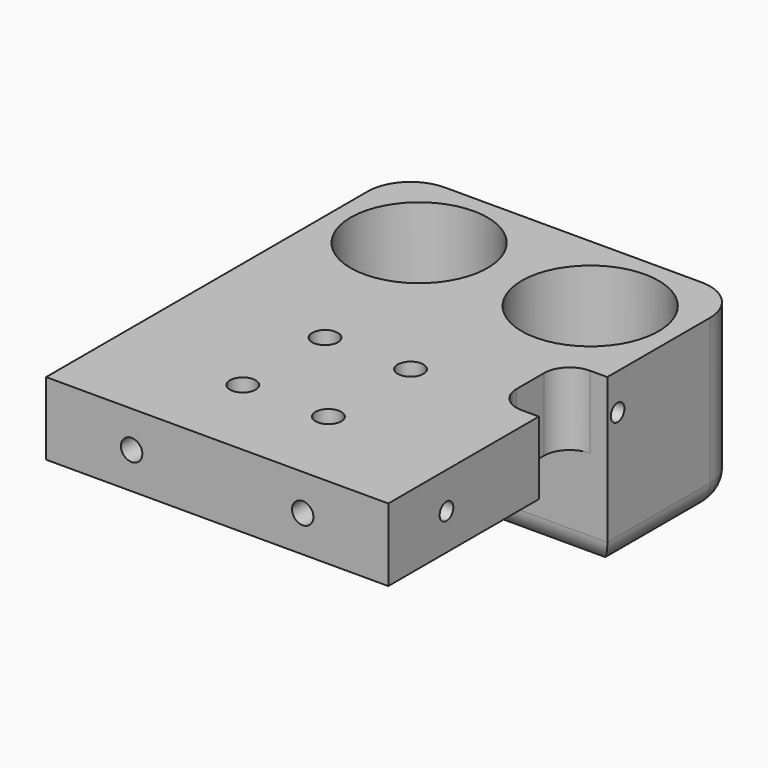
from build123d import *

# Parameters (mm, degrees)
F0_W          = 20
F0_H          = 20
F1_DEPTH      = 20
F2_D          = 3
F2_DEPTH      = 20
F2_TIP        = 0.9012909285
F3_D          = 16
F3_DEPTH      = 20
F3_TIP        = 4.8068849522
F4_W          = 40
F4_H          = 32
F4_R          = 1.5
F5_DEPTH      = 11.5
F7_D          = 2.5
F7_DEPTH      = 5
F7_TIP        = 0.7510757738
F8_R          = 5
F10_D         = 2.5
F10_DEPTH     = 5
F10_TIP       = 0.7510757738
F11_T1_DEPTH  = 22.5
F11_T3_DEPTH  = 55
F11_T5_DEPTH  = 30
F11_T8_ANGLE  = 90
F11_T10_ANGLE = 90
F13_W         = 5
F13_H         = 10
F14_DEPTH     = 25
F15_R         = 3
F16_D         = 2
F16_DEPTH     = 5
F16_TIP       = 0.600860619


# Not quite as in the source:
# - a fillet or chamfer that OpenCascade refuses, or shapes differently, is made with other operations: its cross-section is extruded or revolved along the edge and cut away or added


with BuildPart() as f1:
    # F0 (on Top) → F1 (new body)
    with BuildSketch(Plane.XY):
        with Locations((-5, 20)):
            Rectangle(F0_W, F0_H)
        with Locations((15, 20)):
            Rectangle(F0_W, F0_H)
        Polygon((5, 10), (-15, 10), (-15, -22), (25, -22), (25, 10), align=None)
    extrude(amount=-F1_DEPTH)

    # F2
    with Locations(Plane.XY):
        with Locations((10, 0), (0, 0), (0, -12), (10, -12)):
            Hole(F2_D / 2, depth=F2_DEPTH)
            with Locations((0, 0, -(F2_DEPTH + F2_TIP / 2))):  # 118° drill point
                Cone(0, F2_D / 2, F2_TIP, mode=Mode.SUBTRACT)

    # F3
    with Locations(Plane.XY):
        with Locations((15, 20), (-5, 20)):
            Hole(F3_D / 2, depth=F3_DEPTH)
            with Locations((0, 0, -(F3_DEPTH + F3_TIP / 2))):  # 118° drill point
                Cone(0, F3_D / 2, F3_TIP, mode=Mode.SUBTRACT)

    # F4 (on face) → F5 (cut)
    with BuildSketch(Plane(origin=(0, 0, -20), x_dir=(1, 0, 0), z_dir=(0, 0, -1))):
        with Locations((5, 6)):
            Rectangle(F4_W, F4_H)
        Circle(F4_R, mode=Mode.SUBTRACT)
        with Locations((0, 12)):
            Circle(F4_R, mode=Mode.SUBTRACT)
        with Locations((10, 0)):
            Circle(F4_R, mode=Mode.SUBTRACT)
        with Locations((10, 12)):
            Circle(F4_R, mode=Mode.SUBTRACT)
    extrude(amount=-F5_DEPTH, mode=Mode.SUBTRACT)

    # F7
    with Locations(Plane.XZ.offset(22)):
        with Locations((-5, -4.25), (15, -4.25)):
            Hole(F7_D / 2, depth=F7_DEPTH)
            with Locations((0, 0, -(F7_DEPTH + F7_TIP / 2))):  # 118° drill point
                Cone(0, F7_D / 2, F7_TIP, mode=Mode.SUBTRACT)

    # F8
    f8_edges = [f1.edges().sort_by_distance(p)[0] for p in [
        (-15, 30, -10),
        (25, 30, -10),
    ]]
    fillet(f8_edges, radius=F8_R)

    # F10
    with Locations(Plane(origin=(0, 30, 0), x_dir=(-1, 0, 0), z_dir=(0, 1, 0))):
        with Locations((5, -10), (-15, -10)):
            Hole(F10_D / 2, depth=F10_DEPTH)
            with Locations((0, 0, -(F10_DEPTH + F10_TIP / 2))):  # 118° drill point
                Cone(0, F10_D / 2, F10_TIP, mode=Mode.SUBTRACT)

    # F11: fillet of radius 3 on 2 edges, made by hand

    # F11_s2 → F11_t1 (cut)
    with BuildSketch(Plane.XZ.offset(-25)):
        with BuildLine():
            ThreePointArc((-15, -17), (-14.1213203436, -19.1213203436), (-12, -20))
            Line((-12, -20), (-15, -20))
            Line((-15, -20), (-15, -17))
        make_face()
        with BuildLine():
            ThreePointArc((22, -20), (24.1213203436, -19.1213203436), (25, -17))
            Line((25, -17), (25, -20))
            Line((25, -20), (22, -20))
        make_face()
    extrude(amount=F11_T1_DEPTH, mode=Mode.SUBTRACT)

    # F11_s4 → F11_t3 (cut)
    with BuildSketch(Plane.YZ.offset(-22.5)):
        with BuildLine():
            ThreePointArc((13, -20), (10.8786796564, -19.1213203436), (10, -17))
            Line((10, -17), (10, -20))
            Line((10, -20), (13, -20))
        make_face()
    extrude(amount=F11_T3_DEPTH, mode=Mode.SUBTRACT)

    # F11_s6 → F11_t5 (cut)
    with BuildSketch(Plane.YZ.offset(-10)):
        with BuildLine():
            ThreePointArc((27, -20), (29.1213203436, -19.1213203436), (30, -17))
            Line((30, -17), (30, -20))
            Line((30, -20), (27, -20))
        make_face()
    extrude(amount=F11_T5_DEPTH, mode=Mode.SUBTRACT)

    # F11_s7 → F11_t8 (revolve, cut)
    with BuildSketch(Plane.XZ.offset(-25)):
        with BuildLine():
            ThreePointArc((-15, -17), (-14.1213203436, -19.1213203436), (-12, -20))
            Line((-12, -20), (-15, -20))
            Line((-15, -20), (-15, -17))
        make_face()
    revolve(axis=Axis((-10, 25, -20), (0, 0, -1)), revolution_arc=F11_T8_ANGLE, mode=Mode.SUBTRACT)

    # F11_s9 → F11_t10 (revolve, cut)
    with BuildSketch(Plane.YZ.offset(20)):
        with BuildLine():
            ThreePointArc((27, -20), (29.1213203436, -19.1213203436), (30, -17))
            Line((30, -17), (30, -20))
            Line((30, -20), (27, -20))
        make_face()
    revolve(axis=Axis((20, 25, -20), (0, 0, -1)), revolution_arc=F11_T10_ANGLE, mode=Mode.SUBTRACT)

    # F13 (on face) → F14 (cut)
    with BuildSketch(Plane.XY):
        with Locations((22.5, 5)):
            Rectangle(F13_W, F13_H)
    extrude(amount=-F14_DEPTH, mode=Mode.SUBTRACT)

    # F15
    f15_edges = [f1.edges().sort_by_distance(p)[0] for p in [
        (20, 10, -4.25),
        (20, 0, -4.25),
    ]]
    fillet(f15_edges, radius=F15_R)

    # F16
    with Locations(Plane.YZ.offset(25)):
        with Locations((-13.5, -4.25), (11.5, -4.25)):
            Hole(F16_D / 2, depth=F16_DEPTH)
            with Locations((0, 0, -(F16_DEPTH + F16_TIP / 2))):  # 118° drill point
                Cone(0, F16_D / 2, F16_TIP, mode=Mode.SUBTRACT)


solid = f1.part
